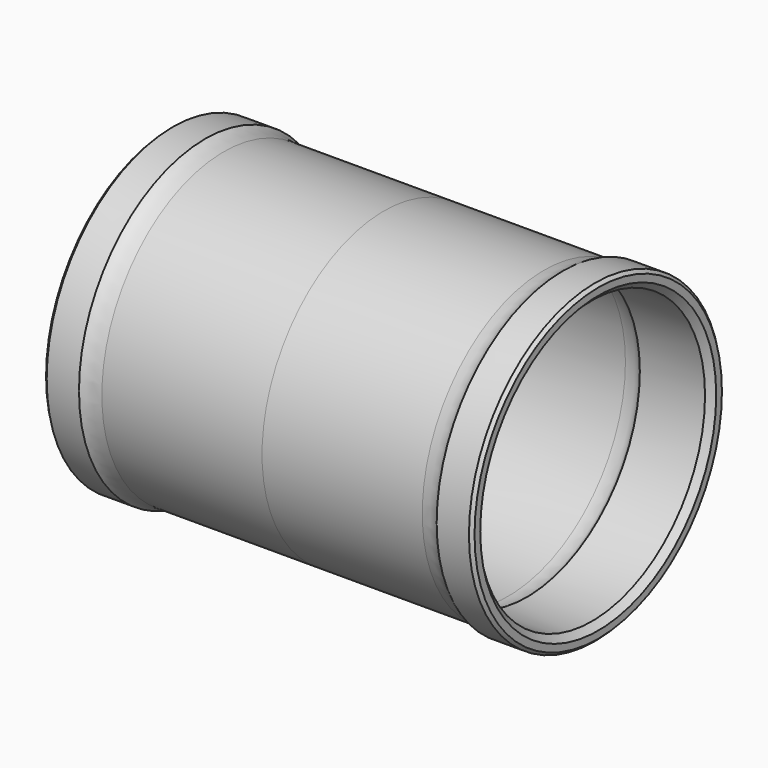
from build123d import *

# Parameters (mm, degrees)
F2_SIZE = 0.5
F3_SIZE = 1


with BuildPart() as f1:
    # F0 (on Top) → F1 (revolve)
    with BuildSketch(Plane.XY):
        with BuildLine():
            Line((-34.5, 25.4), (-34.5, 22.75))
            Line((-34.5, 22.75), (-25.8, 22.75))
            Line((-25.8, 22.75), (-23, 22.75))
            add(Edge.make_bspline(
                [(-23, 22.75), (-22.4767401814, 23.4261993319), (-21.5331446379, 23.6), (-20, 23.6)],
                knots=[0, 0, 0, 0, 3.1180923655, 3.1180923655, 3.1180923655, 3.1180923655], degree=3))
            Line((-20, 23.6), (0, 23.6))
            Line((0, 23.6), (0, 24.55))
            Line((0, 24.55), (-25.8, 24.55))
            add(Edge.make_bspline(
                [(-28.8, 25.4), (-28.3960923553, 25.0019170344), (-27.5980718434, 24.6472395957), (-25.8, 24.55)],
                knots=[0, 0, 0, 0, 3.1180923655, 3.1180923655, 3.1180923655, 3.1180923655], degree=3))
            Line((-28.8, 25.4), (-34.5, 25.4))
        make_face()
    revolve(axis=Axis((-33.9306145906, 0, 0), (-1, 0, 0)))

    # F2
    f2_edges = [f1.edges().sort_by_distance(p)[0] for p in [
        (-34.5, -25.4, 0),
    ]]
    chamfer(f2_edges, length=F2_SIZE)

    # F3
    f3_edges = [f1.edges().sort_by_distance(p)[0] for p in [
        (-34.5, -22.75, 0),
    ]]
    chamfer(f3_edges, length=F3_SIZE)

    # F4: F1 across face


with BuildPart() as f1_1:
    add(f1.part)
    add(f1.part.mirror(Plane.YZ))


solid = f1_1.part
